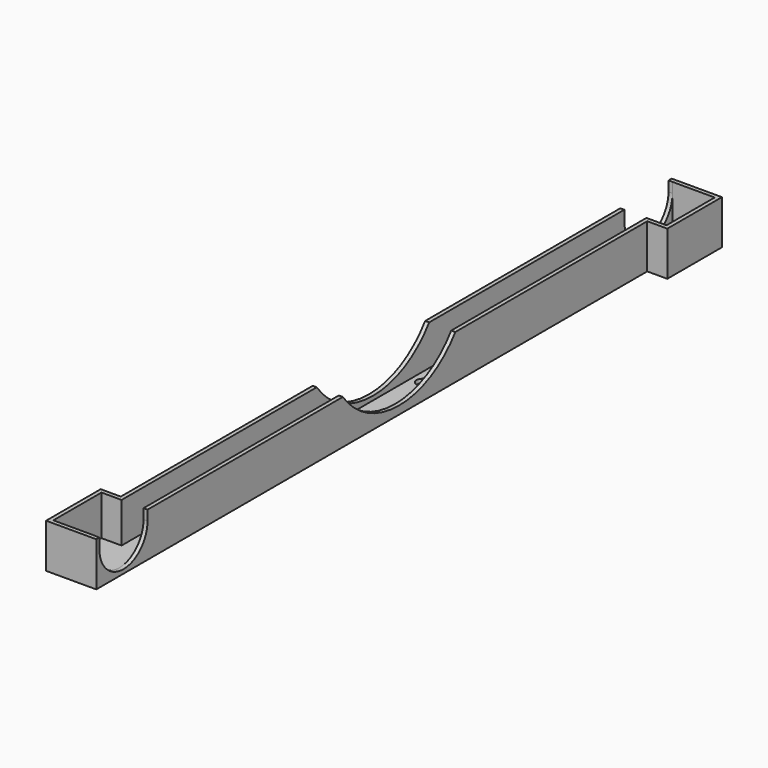
from build123d import *

# Parameters (mm, degrees)
F1_DEPTH = 22
F3_DEPTH = 20
F5_DEPTH = 2
F6_DEPTH = 2
F7_DEPTH = 22
F9_DEPTH = 15


# Not quite as in the source:
# - a feature names something its author has since deleted; it is built from what else it names


with BuildPart() as f1:
    # F0 (on Top) → F1 (new body)
    with BuildSketch(Plane.XY):
        Polygon((-13, 345), (-13, 156.5), (-13, 2), (-23, 2), (-23, -32), (2, -32), (2, 311), (12, 311), (12, 345), align=None)
        Polygon((10, 313), (0, 313), (0, -30), (-21, -30), (-21, 0), (-11, 0), (-11, 156.5), (-11, 343), (10, 343), align=None, mode=Mode.SUBTRACT)
        Polygon((0, -30), (0, 313), (10, 313), (10, 343), (-11, 343), (-11, 156.5), (-11, 0), (-21, 0), (-21, -30), align=None)
        with BuildLine():
            ThreePointArc((-2.4999999702, 132.5), (-7.6213203138, 130.3786796564), (-5.4999999702, 135.5))
            ThreePointArc((-5.4999999702, 135.5), (-3.3786796266, 134.6213203436), (-2.4999999702, 132.5))
        make_face(mode=Mode.SUBTRACT)
        with BuildLine():
            ThreePointArc((-2.4999999702, 180.5), (-3.3786796266, 178.3786796564), (-5.4999999702, 177.5))
            ThreePointArc((-5.4999999702, 177.5), (-7.6213203138, 182.6213203436), (-2.4999999702, 180.5))
        make_face(mode=Mode.SUBTRACT)
    extrude(amount=-F1_DEPTH)

    # F0 (on Top) → F3 (cut)
    with BuildSketch(Plane.XY):
        Polygon((0, -30), (0, 313), (10, 313), (10, 343), (-11, 343), (-11, 156.5), (-11, 0), (-21, 0), (-21, -30), align=None)
        with BuildLine():
            ThreePointArc((-2.4999999702, 132.5), (-7.6213203138, 130.3786796564), (-5.4999999702, 135.5))
            ThreePointArc((-5.4999999702, 135.5), (-3.3786796266, 134.6213203436), (-2.4999999702, 132.5))
        make_face(mode=Mode.SUBTRACT)
        with BuildLine():
            ThreePointArc((-2.4999999702, 180.5), (-3.3786796266, 178.3786796564), (-5.4999999702, 177.5))
            ThreePointArc((-5.4999999702, 177.5), (-7.6213203138, 182.6213203436), (-2.4999999702, 180.5))
        make_face(mode=Mode.SUBTRACT)
    extrude(amount=-F3_DEPTH, mode=Mode.SUBTRACT)

    # F4 (on face) → F5 (cut)
    with BuildSketch(Plane.YZ.offset(2)):
        with BuildLine():
            Line((-0.1, 0), (-30.1, 0))
            Line((-30.1, 0), (-30.1, -5))
            ThreePointArc((-30.1, -5), (-15.1, -20), (-0.1, -5))
            Line((-0.1, -5), (-0.1, 0))
        make_face()
    extrude(amount=-F5_DEPTH, mode=Mode.SUBTRACT)

    # F2 (on face) → F6 (cut)
    with BuildSketch(Plane(origin=(-13, 0, 0), x_dir=(0, -1, 0), z_dir=(-1, 0, 0))):
        with BuildLine():
            Line((-343.0150201633, 0), (-343, -5))
            ThreePointArc((-343, -5), (-328.0000676811, -19.9549397135), (-313.0001353623, -5))
            Line((-313.0001353623, -5), (-313.0001353623, 0))
            Line((-313.0001353623, 0), (-343.0150201633, 0))
        make_face()
    extrude(amount=-F6_DEPTH, mode=Mode.SUBTRACT)

    # F0 (on Top) → F7 (cut)
    with BuildSketch(Plane.XY):
        with BuildLine():
            ThreePointArc((-2.4999999702, 180.5), (-7.6213203138, 182.6213203436), (-5.4999999702, 177.5))
            ThreePointArc((-5.4999999702, 177.5), (-3.3786796266, 178.3786796564), (-2.4999999702, 180.5))
        make_face()
    extrude(amount=-F7_DEPTH, mode=Mode.SUBTRACT)

    # F8 (on face) → F9 (cut)
    with BuildSketch(Plane(origin=(-13, 0, 0), x_dir=(0, -1, 0), z_dir=(-1, 0, 0))):
        with BuildLine():
            ThreePointArc((-191.5000676811, 0), (-156.5000676811, -18), (-121.5000676811, 0))
            Line((-121.5000676811, 0), (-156.5000676811, 0))
            Line((-156.5000676811, 0), (-191.5000676811, 0))
        make_face()
    extrude(amount=-F9_DEPTH, mode=Mode.SUBTRACT)


solid = f1.part
